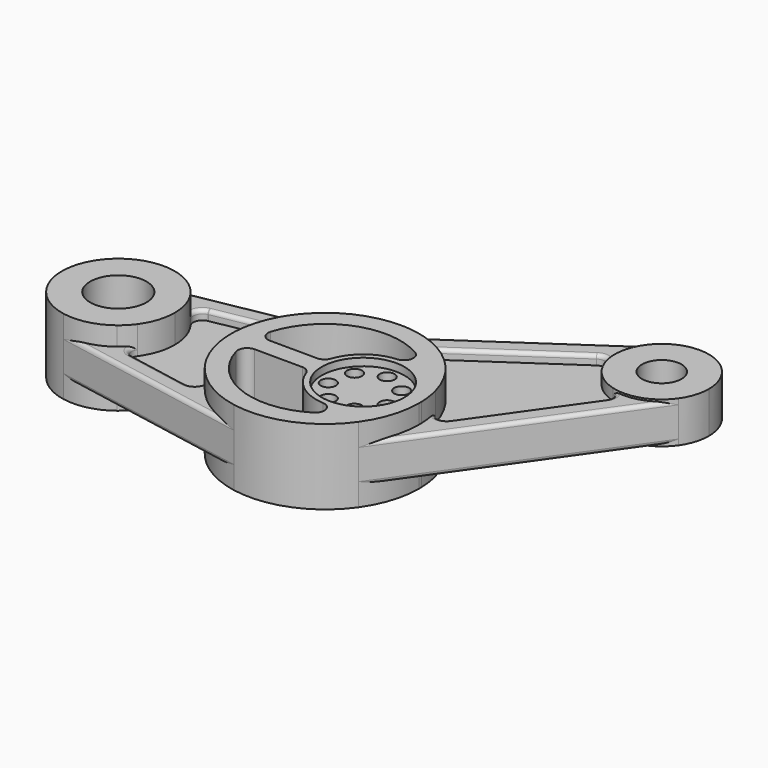
from build123d import *

# Parameters (mm, degrees)
F0_R     = 15
F1_DEPTH = 20
F0_R_2   = 22
F0_R_3   = 4
F2_DEPTH = 16
F3_DEPTH = 20
F4_DEPTH = 10
F0_R_4   = 10.5
F5_DEPTH = 11
F6_DEPTH = 5
F7_R     = 2
F8_R     = 2


with BuildPart() as f1:
    # F0 (on Top) → F1 (new body, symmetric)
    with BuildSketch(Plane.XY):
        with BuildLine():
            ThreePointArc((-111.639854, 23.574294), (-122.9255, 29.002601), (-135.443935, 29.350599))
            ThreePointArc((-135.443935, 29.350599), (-159.999998, -0.140361), (-135.465498, -29.649263))
            ThreePointArc((-135.465498, -29.649263), (-122.946812, -29.310416), (-111.657201, -23.890359))
            ThreePointArc((-111.657201, -23.890359), (-108.452779, -21.025167), (-105.690737, -17.73142))
            ThreePointArc((-105.690737, -17.73142), (-101.458119, -9.39043), (-100, -0.151325))
            ThreePointArc((-100, -0.151325), (-101.455052, 9.078297), (-105.679062, 17.412615))
            ThreePointArc((-105.679062, 17.412615), (-108.438221, 20.707478), (-111.639854, 23.574294))
        make_face()
        with Locations((-130, -0.151325)):
            Circle(F0_R, mode=Mode.SUBTRACT)
    extrude(amount=F1_DEPTH, both=True)


with BuildPart() as f2:
    # F0 (on Top) → F2 (new body, symmetric)
    with BuildSketch(Plane.XY):
        Circle(F0_R_2)
        with Locations((-6.952926, -14.4379)):
            Circle(F0_R_3, mode=Mode.SUBTRACT)
        with Locations((6.952926, -14.4379)):
            Circle(F0_R_3, mode=Mode.SUBTRACT)
        with Locations((-15.623083, -3.565867)):
            Circle(F0_R_3, mode=Mode.SUBTRACT)
        with Locations((-12.52874, 9.991337)):
            Circle(F0_R_3, mode=Mode.SUBTRACT)
        with Locations((15.623083, -3.565867)):
            Circle(F0_R_3, mode=Mode.SUBTRACT)
        with Locations((12.52874, 9.991337)):
            Circle(F0_R_3, mode=Mode.SUBTRACT)
        with Locations((0, 16.02486)):
            Circle(F0_R_3, mode=Mode.SUBTRACT)
    extrude(amount=F2_DEPTH, both=True)

    # F0 (on Top) → F3 (join, symmetric)
    with BuildSketch(Plane.XY):
        with BuildLine():
            ThreePointArc((-29.112634, -49.354756), (-1.158416, -46.504202), (20.844052, -29.02692))
            ThreePointArc((20.844052, -29.02692), (27.653513, -15.318058), (29.99653, -0.191526))
            ThreePointArc((29.99653, -0.191526), (29.991343, 0.528647), (29.975784, 1.248672))
            ThreePointArc((29.975784, 1.248672), (29.453109, 7.160126), (28.233719, 12.968016))
            ThreePointArc((28.233719, 12.968016), (15.640347, 34.872961), (-6.055311, 47.823564))
            ThreePointArc((-6.055311, 47.823564), (-11.84244, 49.137954), (-17.744537, 49.75742))
            ThreePointArc((-17.744537, 49.75742), (-39.030984, 46.046485), (-56.763976, 33.700438))
            ThreePointArc((-56.763976, 33.700438), (-60.520604, 29.106287), (-63.706452, 24.099406))
            ThreePointArc((-63.706452, 24.099406), (-70.003467, -0.173253), (-63.724196, -24.450507))
            ThreePointArc((-63.724196, -24.450507), (-60.542009, -29.459716), (-56.788739, -34.056612))
            ThreePointArc((-56.788739, -34.056612), (-44.19196, -43.95129), (-29.112634, -49.354756))
        make_face()
        with BuildLine():
            ThreePointArc((-58.389802, -11.438283), (-57.58577, -7.024801), (-53.566312, -5.032502))
            Line((-53.566312, -5.032502), (-28.201899, -5.16033))
            ThreePointArc((-28.201899, -5.16033), (-25.341636, -6.076871), (-23.522581, -8.466889))
            ThreePointArc((-23.522581, -8.466889), (-14.913705, -20.064431), (-1.326856, -24.964764))
            ThreePointArc((-1.326856, -24.964764), (3.25182, -28.718679), (1.037951, -34.21003))
            ThreePointArc((1.037951, -34.21003), (-34.316038, -37.543238), (-58.389802, -11.438283))
        make_face(mode=Mode.SUBTRACT)
        with BuildLine():
            ThreePointArc((-58.281465, 11.418604), (-34.496451, 37.090554), (0.382722, 34.223633))
            ThreePointArc((0.382722, 34.223633), (2.701331, 28.775679), (-1.804626, 24.934781))
            ThreePointArc((-1.804626, 24.934781), (-15.217468, 19.835036), (-23.616782, 8.200464))
            ThreePointArc((-23.616782, 8.200464), (-25.452179, 5.758929), (-28.365336, 4.840621))
            Line((-28.365336, 4.840621), (-53.521914, 4.967401))
            ThreePointArc((-53.521914, 4.967401), (-57.520197, 6.998904), (-58.281465, 11.418604))
        make_face(mode=Mode.SUBTRACT)
        Circle(F0_R_2, mode=Mode.SUBTRACT)
    extrude(amount=F3_DEPTH, both=True)


with BuildPart() as f4:
    # F0 (on Top) → F4 (new body, symmetric)
    with BuildSketch(Plane.XY):
        with BuildLine():
            ThreePointArc((55.175907, 99.46396), (58.317645, 110.513643), (66.06927, 118.991752))
            Line((66.06927, 118.991752), (-37.357979, 48.490115))
            ThreePointArc((-37.357979, 48.490115), (-39.550309, 47.308476), (-41.939338, 46.604829))
            Line((-41.939338, 46.604829), (-135.443935, 29.350599))
            ThreePointArc((-135.443935, 29.350599), (-122.9255, 29.002601), (-111.639854, 23.574294))
            Line((-111.639854, 23.574294), (-102.67519, 25.228527))
            ThreePointArc((-102.67519, 25.228527), (-102.532895, 25.256925), (-102.389837, 25.281183))
            Line((-102.389837, 25.281183), (-68.984073, 31.445486))
            Line((-68.984073, 31.445486), (-56.763976, 33.700438))
            ThreePointArc((-56.763976, 33.700438), (-39.030984, 46.046485), (-17.744537, 49.75742))
            Line((-17.744537, 49.75742), (-7.476717, 56.756524))
            Line((-7.476717, 56.756524), (48.330694, 94.797891))
            Line((48.330694, 94.797891), (55.175907, 99.46396))
        make_face()
        with BuildLine():
            ThreePointArc((-63.706452, 24.099406), (-60.520604, 29.106287), (-56.763976, 33.700438))
            Line((-56.763976, 33.700438), (-68.984073, 31.445486))
            ThreePointArc((-68.984073, 31.445486), (-64.016051, 29.445813), (-63.706452, 24.099406))
        make_face()
        with BuildLine():
            Line((-102.67519, 25.228527), (-111.639854, 23.574294))
            ThreePointArc((-111.639854, 23.574294), (-108.438221, 20.707478), (-105.679062, 17.412615))
            ThreePointArc((-105.679062, 17.412615), (-106.29275, 22.133664), (-102.67519, 25.228527))
        make_face()
        with BuildLine():
            ThreePointArc((-6.055311, 47.823564), (-9.598375, 51.839361), (-7.476717, 56.756524))
            Line((-7.476717, 56.756524), (-17.744537, 49.75742))
            ThreePointArc((-17.744537, 49.75742), (-11.84244, 49.137954), (-6.055311, 47.823564))
        make_face()
        with BuildLine():
            ThreePointArc((55.980827, 91.944448), (55.292392, 95.673592), (55.175907, 99.46396))
            Line((55.175907, 99.46396), (48.330694, 94.797891))
            ThreePointArc((48.330694, 94.797891), (52.894286, 95.351169), (55.980827, 91.944448))
        make_face()
    extrude(amount=F4_DEPTH, both=True)

    # F8 (call 1 of 13: OpenCascade refuses the feature's edges together)
    f8_edges = [f4.edges().sort_by_distance(p)[0] for p in [
        (52.894286, 95.351169, 10),
        (20.426988, 75.777208, 10),
        (-9.598375, 51.839361, 10),
    ]]
    fillet(f8_edges, radius=F8_R)

    # F8#2 (call 2 of 13)
    f8_2_edges = [f4.edges().sort_by_distance(p)[0] for p in [
        (-106.238736, 22.268337, -10),
        (-64.016051, 29.445813, -10),
        (-85.686955, 28.363335, -10),
    ]]
    fillet(f8_2_edges, radius=F8_R)

    # F8#3 (call 3 of 13)
    f8_3_edges = [f4.edges().sort_by_distance(p)[0] for p in [
        (-85.686955, 28.363335, 10),
        (-64.016051, 29.445813, 10),
        (-106.238736, 22.268337, 10),
    ]]
    fillet(f8_3_edges, radius=F8_R)

    # F8#4 (call 4 of 13)
    f8_4_edges = [f4.edges().sort_by_distance(p)[0] for p in [
        (-9.598375, 51.839361, -10),
        (20.426988, 75.777208, -10),
        (52.894286, 95.351169, -10),
    ]]
    fillet(f8_4_edges, radius=F8_R)

    # F8#5 (call 5 of 13)
    f8_5_edges = [f4.edges().sort_by_distance(p)[0] for p in [
        (-88.691637, 37.977714, 10),
        (14.355645, 83.740933, 10),
        (-39.550309, 47.308476, 10),
    ]]
    fillet(f8_5_edges, radius=F8_R)

    # F8#6 (call 6 of 13)
    f8_6_edges = [f4.edges().sort_by_distance(p)[0] for p in [
        (14.355645, 83.740933, -10),
        (-88.691637, 37.977714, -10),
        (-39.550309, 47.308476, -10),
    ]]
    fillet(f8_6_edges, radius=F8_R)


with BuildPart() as f4b:
    # F0 (on Top) → F4, piece 2 (new body, symmetric)
    with BuildSketch(Plane.XY):
        with BuildLine():
            Line((20.844052, -29.02692), (100.574141, 83.916797))
            ThreePointArc((100.574141, 83.916797), (91.970157, 76.30513), (80.870479, 73.344867))
            Line((80.870479, 73.344867), (76.092875, 66.577028))
            Line((76.092875, 66.577028), (37.142191, 11.40043))
            Line((37.142191, 11.40043), (29.975784, 1.248672))
            ThreePointArc((29.975784, 1.248672), (29.991343, 0.528647), (29.99653, -0.191526))
            ThreePointArc((29.99653, -0.191526), (27.653513, -15.318058), (20.844052, -29.02692))
        make_face()
        with BuildLine():
            Line((29.975784, 1.248672), (37.142191, 11.40043))
            ThreePointArc((37.142191, 11.40043), (32.190923, 9.359627), (28.233719, 12.968016))
            ThreePointArc((28.233719, 12.968016), (29.453109, 7.160126), (29.975784, 1.248672))
        make_face()
        with BuildLine():
            Line((76.092875, 66.577028), (80.870479, 73.344867))
            ThreePointArc((80.870479, 73.344867), (77.082529, 73.523442), (73.365166, 74.272888))
            ThreePointArc((73.365166, 74.272888), (76.720855, 71.130941), (76.092875, 66.577028))
        make_face()
    extrude(amount=F4_DEPTH, both=True)

    # F8#7 (call 7 of 13)
    f8_7_edges = [f4b.edges().sort_by_distance(p)[0] for p in [
        (76.720855, 71.130941, -10),
        (56.617533, 38.988729, -10),
        (32.190923, 9.359627, -10),
    ]]
    fillet(f8_7_edges, radius=F8_R)

    # F8#8 (call 8 of 13)
    f8_8_edges = [f4b.edges().sort_by_distance(p)[0] for p in [
        (60.709097, 27.444938, -10),
    ]]
    fillet(f8_8_edges, radius=F8_R)

    # F8#9 (call 9 of 13)
    f8_9_edges = [f4b.edges().sort_by_distance(p)[0] for p in [
        (76.720855, 71.130941, 10),
        (32.190923, 9.359627, 10),
        (56.617533, 38.988729, 10),
    ]]
    fillet(f8_9_edges, radius=F8_R)

    # F8#10 (call 10 of 13)
    f8_10_edges = [f4b.edges().sort_by_distance(p)[0] for p in [
        (60.709097, 27.444938, 10),
    ]]
    fillet(f8_10_edges, radius=F8_R)


with BuildPart() as f4c:
    # F0 (on Top) → F4, piece 3 (new body, symmetric)
    with BuildSketch(Plane.XY):
        with BuildLine():
            Line((-135.465498, -29.649263), (-29.112634, -49.354756))
            ThreePointArc((-29.112634, -49.354756), (-44.19196, -43.95129), (-56.788739, -34.056612))
            Line((-56.788739, -34.056612), (-69.007185, -31.792728))
            Line((-69.007185, -31.792728), (-102.550109, -25.577758))
            Line((-102.550109, -25.577758), (-111.657201, -23.890359))
            ThreePointArc((-111.657201, -23.890359), (-122.946812, -29.310416), (-135.465498, -29.649263))
        make_face()
        with BuildLine():
            ThreePointArc((-105.690737, -17.73142), (-108.452779, -21.025167), (-111.657201, -23.890359))
            Line((-111.657201, -23.890359), (-102.550109, -25.577758))
            ThreePointArc((-102.550109, -25.577758), (-106.281149, -22.519456), (-105.690737, -17.73142))
        make_face()
        with BuildLine():
            Line((-69.007185, -31.792728), (-56.788739, -34.056612))
            ThreePointArc((-56.788739, -34.056612), (-60.542009, -29.459716), (-63.724196, -24.450507))
            ThreePointArc((-63.724196, -24.450507), (-64.037703, -29.796687), (-69.007185, -31.792728))
        make_face()
    extrude(amount=F4_DEPTH, both=True)

    # F7
    f7_edges = [f4c.edges().sort_by_distance(p)[0] for p in [
        (-82.289066, -39.502009, 10),
    ]]
    fillet(f7_edges, radius=F7_R)

    # F8#11 (call 11 of 13)
    f8_11_edges = [f4c.edges().sort_by_distance(p)[0] for p in [
        (-106.281149, -22.519456, 10),
        (-64.037703, -29.796687, 10),
        (-85.778647, -28.685243, 10),
    ]]
    fillet(f8_11_edges, radius=F8_R)

    # F8#12 (call 12 of 13)
    f8_12_edges = [f4c.edges().sort_by_distance(p)[0] for p in [
        (-82.289066, -39.502009, -10),
    ]]
    fillet(f8_12_edges, radius=F8_R)

    # F8#13 (call 13 of 13)
    f8_13_edges = [f4c.edges().sort_by_distance(p)[0] for p in [
        (-106.281149, -22.519456, -10),
        (-64.037703, -29.796687, -10),
        (-85.778647, -28.685243, -10),
    ]]
    fillet(f8_13_edges, radius=F8_R)


with BuildPart() as f5:
    # F0 (on Top) → F5 (new body, symmetric)
    with BuildSketch(Plane.XY):
        with BuildLine():
            ThreePointArc((100.574141, 83.916797), (103.978872, 90.771228), (105.15038, 98.334494))
            ThreePointArc((105.15038, 98.334494), (91.833108, 120.436844), (66.06927, 118.991752))
            ThreePointArc((66.06927, 118.991752), (58.317645, 110.513643), (55.175907, 99.46396))
            ThreePointArc((55.175907, 99.46396), (55.292392, 95.673592), (55.980827, 91.944448))
            ThreePointArc((55.980827, 91.944448), (62.328472, 80.80225), (73.365166, 74.272888))
            ThreePointArc((73.365166, 74.272888), (77.082529, 73.523442), (80.870479, 73.344867))
            ThreePointArc((80.870479, 73.344867), (91.970157, 76.30513), (100.574141, 83.916797))
        make_face()
        with Locations((80.15038, 98.334494)):
            Circle(F0_R_4, mode=Mode.SUBTRACT)
    extrude(amount=F5_DEPTH, both=True)


with BuildPart() as f6:
    # F0 (on Top) → F6 (new body, symmetric)
    with BuildSketch(Plane.XY):
        with BuildLine():
            ThreePointArc((-69.007185, -31.792728), (-64.037703, -29.796687), (-63.724196, -24.450507))
            ThreePointArc((-63.724196, -24.450507), (-70.003467, -0.173253), (-63.706452, 24.099406))
            ThreePointArc((-63.706452, 24.099406), (-64.016051, 29.445813), (-68.984073, 31.445486))
            Line((-68.984073, 31.445486), (-102.389837, 25.281183))
            Line((-102.389837, 25.281183), (-102.67519, 25.228527))
            ThreePointArc((-102.67519, 25.228527), (-106.29275, 22.133664), (-105.679062, 17.412615))
            ThreePointArc((-105.679062, 17.412615), (-101.455052, 9.078297), (-100, -0.151325))
            ThreePointArc((-100, -0.151325), (-101.458119, -9.39043), (-105.690737, -17.73142))
            ThreePointArc((-105.690737, -17.73142), (-106.281149, -22.519456), (-102.550109, -25.577758))
            Line((-102.550109, -25.577758), (-69.007185, -31.792728))
        make_face()
    extrude(amount=F6_DEPTH, both=True)


with BuildPart() as f6b:
    # F0 (on Top) → F6, piece 2 (new body, symmetric)
    with BuildSketch(Plane.XY):
        with BuildLine():
            ThreePointArc((73.365166, 74.272888), (62.328472, 80.80225), (55.980827, 91.944448))
            ThreePointArc((55.980827, 91.944448), (52.894286, 95.351169), (48.330694, 94.797891))
            Line((48.330694, 94.797891), (-7.476717, 56.756524))
            ThreePointArc((-7.476717, 56.756524), (-9.598375, 51.839361), (-6.055311, 47.823564))
            ThreePointArc((-6.055311, 47.823564), (15.640347, 34.872961), (28.233719, 12.968016))
            ThreePointArc((28.233719, 12.968016), (32.190923, 9.359627), (37.142191, 11.40043))
            Line((37.142191, 11.40043), (76.092875, 66.577028))
            ThreePointArc((76.092875, 66.577028), (76.720855, 71.130941), (73.365166, 74.272888))
        make_face()
    extrude(amount=F6_DEPTH, both=True)


solid = Compound([f1.part, f2.part, f4.part, f4b.part, f4c.part, f5.part, f6.part, f6b.part])
